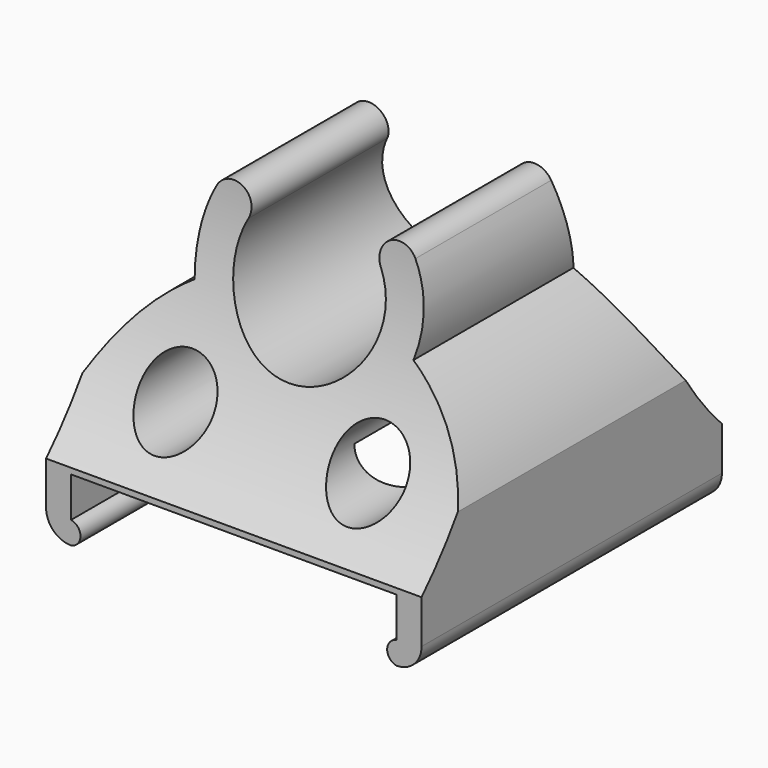
from build123d import *

# Parameters (mm, degrees)
F0_R          = 1.5
F1_DEPTH      = 15
F2_R          = 14.550115737
F3_DEPTH      = 25
F3_DEPTH_BACK = 25
F4_R          = 5
F5_DEPTH      = 3.5


# Not quite as in the source:
# - ends of sketch curves that miss each other by under 0.0002 mm in the source are joined


with BuildPart() as f1:
    # F0 (on Front) → F1 (new body)
    with BuildSketch(Plane.XZ):
        with BuildLine():
            Line((-6.5, -0.8), (-6.5, 0.8))
            Line((-6.5, 0.8), (6.5, 0.8))
            Line((6.5, 0.8), (6.5, -0.8))
            ThreePointArc((6.5, -0.8), (6.1264578545, -1.2499931592), (6.4999470351, -1.7000302796))
            ThreePointArc((6.4999470351, -1.7000302796), (7.2070390333, -1.4071599085), (7.4999451737, -0.7000767547))
            Line((7.4999451737, -0.7000767547), (7.5000913757, 3.3000402053))
            ThreePointArc((7.5000913757, 3.3000402053), (6.2070011857, 5.3492777345), (4.3711160801, 6.93072725))
            ThreePointArc((4.3711160801, 6.93072725), (4.4644607322, 8.5644381014), (3.967454999, 10.1235114388))
            ThreePointArc((3.967454999, 10.1235114388), (2.952293926, 10.4308353655), (2.6449699993, 9.4156742925))
            ThreePointArc((2.6449699993, 9.4156742925), (0, 5), (-2.6449699993, 9.4156742925))
            ThreePointArc((-2.6449699993, 9.4156742925), (-2.952293926, 10.4308353655), (-3.967454999, 10.1235114388))
            ThreePointArc((-3.967454999, 10.1235114388), (-4.4644607322, 8.5644381014), (-4.3711160801, 6.93072725))
            ThreePointArc((-4.3711160801, 6.93072725), (-6.2070011857, 5.3492777345), (-7.5000913757, 3.3000402053))
            Line((-7.5000913757, 3.3000402053), (-7.4999451737, -0.7000767547))
            ThreePointArc((-7.4999451737, -0.7000767547), (-7.2070390333, -1.4071599085), (-6.4999451744, -1.7000402053))
            ThreePointArc((-6.4999451744, -1.7000402053), (-6.1264578541, -1.2500021402), (-6.5, -0.8))
        make_face()
        with Locations((-3.848537337, 3.4744446166)):
            Circle(F0_R, mode=Mode.SUBTRACT)
        with Locations((3.848537337, 3.4744446166)):
            Circle(F0_R, mode=Mode.SUBTRACT)
    extrude(amount=F1_DEPTH)

    # F2 (on Right) → F3 (cut, two sides)
    with BuildSketch(Plane.YZ) as f3_sk:
        with Locations((-25.4004554451, 11.2085361034)):
            Circle(F2_R)
        with Locations((10.4004554451, 11.2085361034)):
            Circle(F2_R)
    extrude(amount=-F3_DEPTH, mode=Mode.SUBTRACT)
    extrude(f3_sk.sketch, amount=F3_DEPTH_BACK, mode=Mode.SUBTRACT)

    # F4 (on Top) → F5 (cut)
    with BuildSketch(Plane.XY):
        with Locations((0, -7.5)):
            Circle(F4_R)
    extrude(amount=F5_DEPTH, mode=Mode.SUBTRACT)


solid = f1.part
